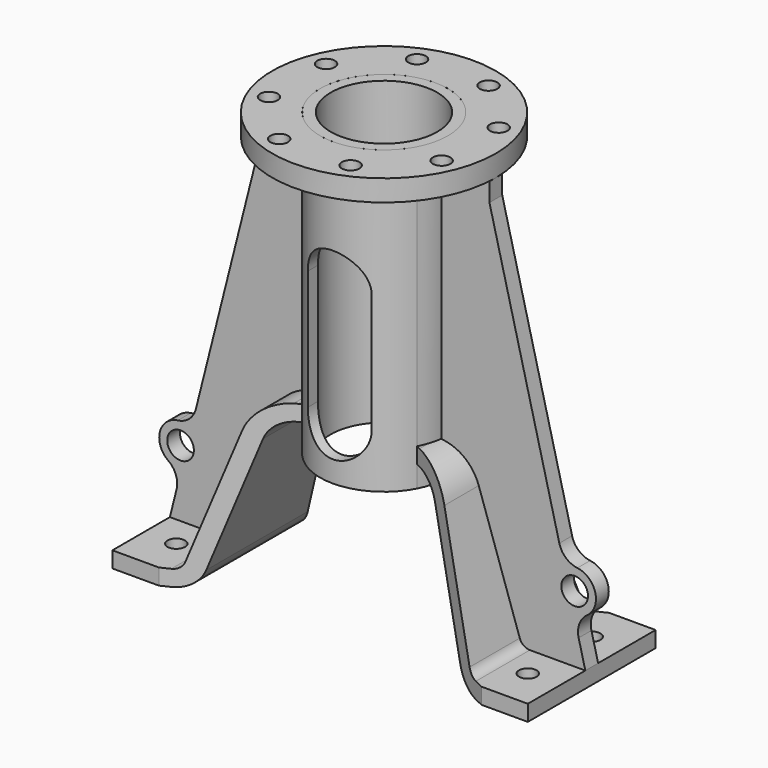
from build123d import *
from build123d import SkipClean  # not in build123d's __all__

# Parameters (mm, degrees)
F2_DEPTH = 30
F4_R     = 3.3
F4_R_2   = 20
F5_DEPTH = 200
F6_DEPTH = 113
F0_R     = 5
F7_DEPTH = 3
F8_DEPTH = 45
F1_R     = 42
F1_R_2   = 3.3
F1_R_3   = 24
F9_DEPTH = 8


with BuildPart() as f2:
    # F0 (on Front) → F2 (new body, symmetric)
    with BuildSketch(Plane.XZ):
        with BuildLine():
            Line((-24, -105.0685745171), (-24, -99.0427692841))
            ThreePointArc((-24, -99.0427692841), (-32.6224560727, -102.3459299934), (-37.9839570353, -109.8633715015))
            Line((-37.9839570353, -109.8633715015), (-53.3808335177, -155.2841571246))
            ThreePointArc((-53.3808335177, -155.2841571246), (-54.8384993115, -157.2508943768), (-57.1690970354, -158))
            Line((-57.1690970354, -158), (-78, -158))
            Line((-78, -158), (-78, -164))
            Line((-78, -164), (-57.1690970354, -164))
            ThreePointArc((-57.1690970354, -164), (-51.3426027256, -162.1272359421), (-47.6984382412, -157.2103928116))
            Line((-47.6984382412, -157.2103928116), (-32.3015617588, -111.7896071884))
            ThreePointArc((-32.3015617588, -111.7896071884), (-29.1232928977, -107.2278813101), (-24, -105.0685745171))
        make_face()
        with BuildLine():
            ThreePointArc((-22.8309029646, -99), (-23.4158425106, -99.0106958961), (-24, -99.0427692841))
            Line((-24, -99.0427692841), (-24, -105.0685745171))
            ThreePointArc((-24, -105.0685745171), (-23.416456195, -105.0171583497), (-22.8309029646, -105))
            Line((-22.8309029646, -105), (-20, -105))
            Line((-20, -105), (-20, -99))
            Line((-20, -99), (-22.8309029646, -99))
        make_face()
        with BuildLine():
            Line((-10.3923048454, -99), (-20, -99))
            Line((-20, -99), (-20, -105))
            Line((-20, -105), (0, -105))
            ThreePointArc((0, -105), (-6, -103.3923048454), (-10.3923048454, -99))
        make_face()
    extrude(amount=F2_DEPTH, both=True)


with BuildPart() as f2b:
    # F0 (on Front) → F2, piece 2 (new body, symmetric)
    with BuildSketch(Plane.XZ):
        with BuildLine():
            ThreePointArc((37.9839570353, -109.8633715015), (32.6224560727, -102.3459299934), (24, -99.0427692841))
            Line((24, -99.0427692841), (24, -105.0685745171))
            ThreePointArc((24, -105.0685745171), (29.1232928977, -107.2278813101), (32.3015617588, -111.7896071884))
            Line((32.3015617588, -111.7896071884), (47.6984382412, -157.2103928116))
            ThreePointArc((47.6984382412, -157.2103928116), (51.3426027256, -162.1272359421), (57.1690970354, -164))
            Line((57.1690970354, -164), (78, -164))
            Line((78, -164), (78, -158))
            Line((78, -158), (57.1690970354, -158))
            ThreePointArc((57.1690970354, -158), (54.8384993115, -157.2508943768), (53.3808335177, -155.2841571246))
            Line((53.3808335177, -155.2841571246), (37.9839570353, -109.8633715015))
        make_face()
        with BuildLine():
            Line((20, -105), (20, -99))
            Line((20, -99), (10.3923048454, -99))
            ThreePointArc((10.3923048454, -99), (6, -103.3923048454), (0, -105))
            Line((0, -105), (20, -105))
        make_face()
        with BuildLine():
            Line((22.8309029646, -99), (20, -99))
            Line((20, -99), (20, -105))
            Line((20, -105), (22.8309029646, -105))
            ThreePointArc((22.8309029646, -105), (23.416456195, -105.0171583497), (24, -105.0685745171))
            Line((24, -105.0685745171), (24, -99.0427692841))
            ThreePointArc((24, -99.0427692841), (23.4158425106, -99.0106958961), (22.8309029646, -99))
        make_face()
    extrude(amount=F2_DEPTH, both=True)


with BuildPart() as f3:
    # F0 (on Front) → F3 (revolve)
    with BuildSketch(Plane.XZ):
        with BuildLine():
            Line((-20, -8), (-24, -8))
            Line((-24, -8), (-24, -99.0427692841))
            ThreePointArc((-24, -99.0427692841), (-23.4158425106, -99.0106958961), (-22.8309029646, -99))
            Line((-22.8309029646, -99), (-20, -99))
            Line((-20, -99), (-20, -8))
        make_face()
        with BuildLine():
            ThreePointArc((-22.8309029646, -99), (-23.4158425106, -99.0106958961), (-24, -99.0427692841))
            Line((-24, -99.0427692841), (-24, -105.0685745171))
            ThreePointArc((-24, -105.0685745171), (-23.416456195, -105.0171583497), (-22.8309029646, -105))
            Line((-22.8309029646, -105), (-20, -105))
            Line((-20, -105), (-20, -99))
            Line((-20, -99), (-22.8309029646, -99))
        make_face()
        with BuildLine():
            ThreePointArc((-22.8309029646, -105), (-23.416456195, -105.0171583497), (-24, -105.0685745171))
            Line((-24, -105.0685745171), (-24, -113))
            Line((-24, -113), (-20, -113))
            Line((-20, -113), (-20, -105))
            Line((-20, -105), (-22.8309029646, -105))
        make_face()
    revolve(axis=Axis((0, 0, -2.4781511165), (0, 0, -1)))


with BuildPart() as f5_tool:
    # F4 (on Top) → F5 (new body)
    with BuildSketch(Plane.XY):
        with BuildLine():
            Line((0, 30), (-60.5552109973, 30))
            Line((-60.5552109973, 30), (-21.2798758432, 11.0980576724))
            ThreePointArc((-21.2798758432, 11.0980576724), (0, 24), (21.2798758432, 11.0980576724))
            Line((21.2798758432, 11.0980576724), (60.5552109973, 30))
            Line((60.5552109973, 30), (0, 30))
        make_face()
        with BuildLine():
            Line((-21.2798758432, -11.0980576724), (-60.5552109973, -30))
            Line((-60.5552109973, -30), (0, -30))
            Line((0, -30), (60.5552109973, -30))
            Line((60.5552109973, -30), (21.2798758432, -11.0980576724))
            ThreePointArc((21.2798758432, -11.0980576724), (0, -24), (-21.2798758432, -11.0980576724))
        make_face()
        with Locations((-66, 15)):
            Circle(F4_R)
        with Locations((-66, -15)):
            Circle(F4_R)
        with Locations((66, 15)):
            Circle(F4_R)
        with Locations((66, -15)):
            Circle(F4_R)
        with BuildLine():
            ThreePointArc((21.2798758432, 11.0980576724), (0, 24), (-21.2798758432, 11.0980576724))
            ThreePointArc((-21.2798758432, 11.0980576724), (-24, 0), (-21.2798758432, -11.0980576724))
            ThreePointArc((-21.2798758432, -11.0980576724), (0, -24), (21.2798758432, -11.0980576724))
            ThreePointArc((21.2798758432, -11.0980576724), (23.310051697, -5.7132731321), (24, 0))
            ThreePointArc((24, 0), (23.310051697, 5.7132731321), (21.2798758432, 11.0980576724))
        make_face()
        Circle(F4_R_2, mode=Mode.SUBTRACT)
        Circle(F4_R_2)
    extrude(amount=-F5_DEPTH)


with BuildPart() as f2_1:
    add(f2.part, clean=False)

    # F5: cut by f5_tool
    add(f5_tool.part, mode=Mode.SUBTRACT)


with BuildPart() as f2b_1:
    add(f2b.part, clean=False)

    # F5: cut by f5_tool
    add(f5_tool.part, mode=Mode.SUBTRACT)


with BuildPart() as f3_1:
    add(f3.part, clean=False)

    # F5: cut by f5_tool
    add(f5_tool.part, mode=Mode.SUBTRACT)


with BuildPart() as f6:
    # F4 (on Top) → F6 (new body)
    with BuildSketch(Plane.XY):
        with BuildLine():
            ThreePointArc((21.2798758432, 11.0980576724), (0, 24), (-21.2798758432, 11.0980576724))
            ThreePointArc((-21.2798758432, 11.0980576724), (-24, 0), (-21.2798758432, -11.0980576724))
            ThreePointArc((-21.2798758432, -11.0980576724), (0, -24), (21.2798758432, -11.0980576724))
            ThreePointArc((21.2798758432, -11.0980576724), (23.310051697, -5.7132731321), (24, 0))
            ThreePointArc((24, 0), (23.310051697, 5.7132731321), (21.2798758432, 11.0980576724))
        make_face()
        Circle(F4_R_2, mode=Mode.SUBTRACT)
    extrude(amount=-F6_DEPTH)

    # F0 (on Front) → F8 (cut, symmetric)
    with BuildSketch(Plane.XZ):
        with BuildLine():
            ThreePointArc((-12, -93), (-11.5911099155, -96.1058285412), (-10.3923048454, -99))
            ThreePointArc((-10.3923048454, -99), (-6, -103.3923048454), (0, -105))
            ThreePointArc((0, -105), (6, -103.3923048454), (10.3923048454, -99))
            ThreePointArc((10.3923048454, -99), (11.5911099155, -96.1058285412), (12, -93))
            Line((12, -93), (12, -48))
            ThreePointArc((12, -48), (8.4852813742, -39.5147186258), (0, -36))
            ThreePointArc((0, -36), (-8.4852813742, -39.5147186258), (-12, -48))
            Line((-12, -48), (-12, -93))
        make_face()
    with SkipClean():  # cleaning this boolean's faces spoils the solid; the shape is the same uncleaned
        extrude(amount=F8_DEPTH, both=True, mode=Mode.SUBTRACT)


with BuildPart() as f7:
    # F0 (on Front) → F7 (new body, symmetric)
    with BuildSketch(Plane.XZ):
        with BuildLine():
            Line((-24, -8), (-42, -8))
            Line((-42, -8), (-42, -15))
            Line((-42, -15), (-68.2361190347, -119.0801085989))
            ThreePointArc((-68.2361190347, -119.0801085989), (-70.6920245528, -123.1158990553), (-74.996727312, -125.0623344322))
            ThreePointArc((-74.996727312, -125.0623344322), (-81.7595464762, -131.0533519878), (-78.6255473359, -139.5271978554))
            ThreePointArc((-78.6255473359, -139.5271978554), (-75.7478185119, -143.2793557346), (-75.4915481955, -148.001043723))
            Line((-75.4915481955, -148.001043723), (-78, -158))
            Line((-78, -158), (-57.1690970354, -158))
            ThreePointArc((-57.1690970354, -158), (-54.8384993115, -157.2508943768), (-53.3808335177, -155.2841571246))
            Line((-53.3808335177, -155.2841571246), (-37.9839570353, -109.8633715015))
            ThreePointArc((-37.9839570353, -109.8633715015), (-32.6224560727, -102.3459299934), (-24, -99.0427692841))
            Line((-24, -99.0427692841), (-24, -8))
        make_face()
        with Locations((-74, -133)):
            Circle(F0_R, mode=Mode.SUBTRACT)
    extrude(amount=F7_DEPTH, both=True)


with BuildPart() as f7b:
    # F0 (on Front) → F7, piece 2 (new body, symmetric)
    with BuildSketch(Plane.XZ):
        with BuildLine():
            Line((42, -15), (42, -8))
            Line((42, -8), (24, -8))
            Line((24, -8), (24, -99.0427692841))
            ThreePointArc((24, -99.0427692841), (32.6224560727, -102.3459299934), (37.9839570353, -109.8633715015))
            Line((37.9839570353, -109.8633715015), (53.3808335177, -155.2841571246))
            ThreePointArc((53.3808335177, -155.2841571246), (54.8384993115, -157.2508943768), (57.1690970354, -158))
            Line((57.1690970354, -158), (78, -158))
            Line((78, -158), (75.4915481955, -148.001043723))
            ThreePointArc((75.4915481955, -148.001043723), (75.7478185119, -143.2793557346), (78.6255473359, -139.5271978554))
            ThreePointArc((78.6255473359, -139.5271978554), (81.7595464762, -131.0533519878), (74.996727312, -125.0623344322))
            ThreePointArc((74.996727312, -125.0623344322), (70.6920245528, -123.1158990553), (68.2361190347, -119.0801085989))
            Line((68.2361190347, -119.0801085989), (42, -15))
        make_face()
        with Locations((74, -133)):
            Circle(F0_R, mode=Mode.SUBTRACT)
    extrude(amount=F7_DEPTH, both=True)


with BuildPart() as f9:
    # F1 (on Top) → F9 (new body)
    with BuildSketch(Plane.XY):
        Circle(F1_R)
        with Locations((-13.3939201328, -32.4730413695)):
            Circle(F1_R_2, mode=Mode.SUBTRACT)
        with Locations((-32.3843115743, -13.5110769349)):
            Circle(F1_R_2, mode=Mode.SUBTRACT)
        with Locations((13.4424480692, -32.4529404401)):
            Circle(F1_R_2, mode=Mode.SUBTRACT)
        with Locations((32.4044125037, -13.4625489986)):
            Circle(F1_R_2, mode=Mode.SUBTRACT)
        with Locations((-32.4044125037, 13.325291267)):
            Circle(F1_R_2, mode=Mode.SUBTRACT)
        with Locations((-13.4424480692, 32.3156827085)):
            Circle(F1_R_2, mode=Mode.SUBTRACT)
        Circle(F1_R_3, mode=Mode.SUBTRACT)
        with Locations((32.3843115743, 13.3738192034)):
            Circle(F1_R_2, mode=Mode.SUBTRACT)
        with Locations((13.3939201328, 32.3357836379)):
            Circle(F1_R_2, mode=Mode.SUBTRACT)
    extrude(amount=-F9_DEPTH)


solid = Compound([f2_1.part, f2b_1.part, f6.part, f7.part, f7b.part, f9.part])
